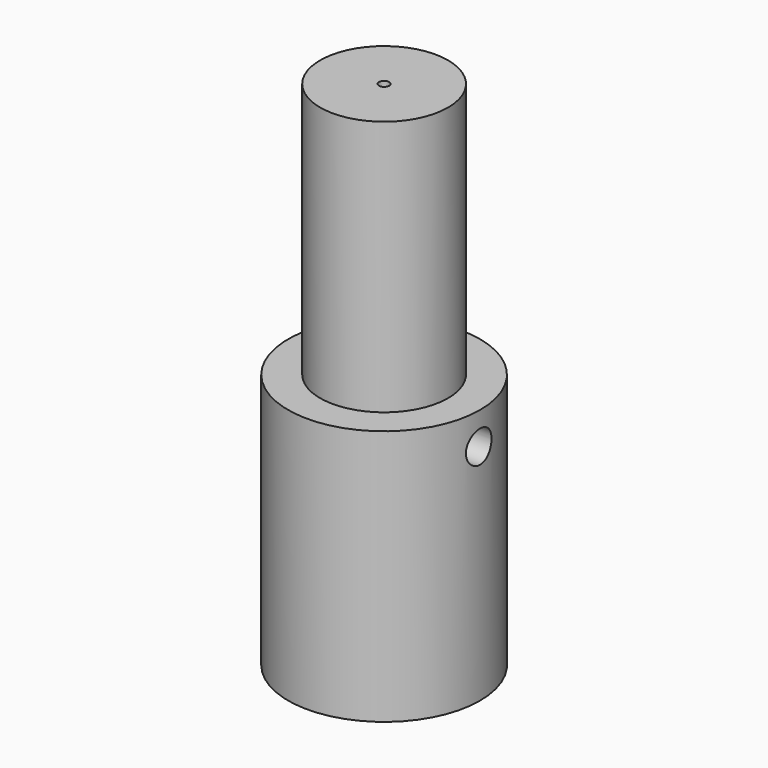
from build123d import *

# Parameters (mm, degrees)
F0_R          = 3.175
F1_DEPTH      = 12.7
F2_R          = 4.7625
F2_R_2        = 3.175
F3_DEPTH      = 12.7
F4_R          = 0.254
F5_DEPTH      = 25.4
F6_R          = 3.7465
F6_R_2        = 0.254
F7_DEPTH      = 6.35
F8_R          = 0.79375
F9_DEPTH      = 4.7635
F9_DEPTH_BACK = 4.7635


with BuildPart() as f1:
    # F0 (on Top) → F1 (new body)
    with BuildSketch(Plane.XY):
        Circle(F0_R)
    extrude(amount=F1_DEPTH)

    # F2 (on face) → F3 (join)
    with BuildSketch(Plane(origin=(0, 0, 0), x_dir=(1, 0, 0), z_dir=(0, 0, -1))):
        Circle(F2_R)
        Circle(F2_R_2, mode=Mode.SUBTRACT)
        Circle(F2_R_2)
    extrude(amount=F3_DEPTH)

    # F4 (on face) → F5 (cut)
    with BuildSketch(Plane(origin=(0, 0, -12.7), x_dir=(1, 0, 0), z_dir=(0, 0, -1))):
        Circle(F4_R)
    extrude(amount=-F5_DEPTH, mode=Mode.SUBTRACT)

    # F6 (on face) → F7 (cut)
    with BuildSketch(Plane(origin=(0, 0, -12.7), x_dir=(1, 0, 0), z_dir=(0, 0, -1))):
        Circle(F6_R)
        Circle(F6_R_2, mode=Mode.SUBTRACT)
    extrude(amount=-F7_DEPTH, mode=Mode.SUBTRACT)

    # F8 (on Right) → F9 (cut, two sides)
    with BuildSketch(Plane.YZ) as f9_sk:
        with Locations((0, -1.6002)):
            Circle(F8_R)
    extrude(amount=-F9_DEPTH, mode=Mode.SUBTRACT)
    extrude(f9_sk.sketch, amount=F9_DEPTH_BACK, mode=Mode.SUBTRACT)


solid = f1.part
